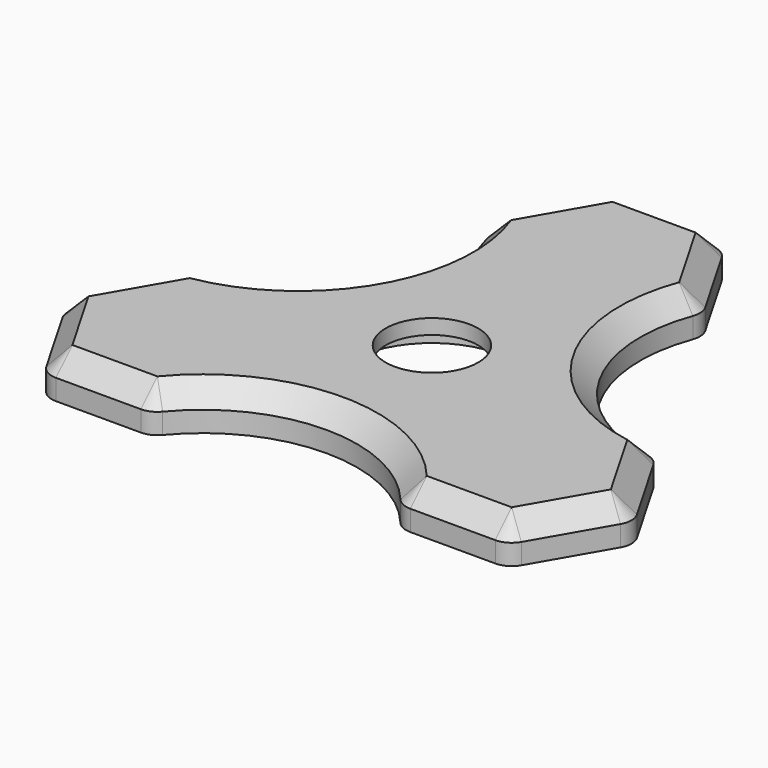
from build123d import *

# Parameters (mm, degrees)
F1_DEPTH = 4
F2_R     = 8.075
F3_DEPTH = 2.55
F5_DEPTH = 3.2
F6_SIZE  = 1.99999
F7_R     = 4.5
F8_DEPTH = 25


# Not quite as in the source:
# - a fillet or chamfer is up to 0.001 mm smaller than in the source, because OpenCascade refuses the exact size


with BuildPart() as f1:
    # F0 (on Top) → F1 (new body)
    with BuildSketch(Plane.XY):
        with BuildLine():
            Line((-5.7735026919, 28), (-9.9042445516, 20.8453452261))
            ThreePointArc((-9.9042445516, 20.8453452261), (-10.1650850266, 20.0138217399), (-10.0475406836, 19.1503100787))
            ThreePointArc((-10.0475406836, 19.1503100787), (-11.1235598668, 6.4221902835), (-21.6084253603, -0.8737295618))
            ThreePointArc((-21.6084253603, -0.8737295618), (-22.4150205669, -1.2036890053), (-23.0047207922, -1.8453452261))
            Line((-23.0047207922, -1.8453452261), (-27.1354626519, -9))
            ThreePointArc((-27.1354626519, -9), (-27.4034118443, -10), (-27.1354626519, -11))
            Line((-27.1354626519, -11), (-23.0940107676, -18))
            ThreePointArc((-23.0940107676, -18), (-22.36195996, -18.7320508076), (-21.36195996, -19))
            Line((-21.36195996, -19), (-13.1004762407, -19))
            ThreePointArc((-13.1004762407, -19), (-12.2499355402, -18.8101327346), (-11.5608846767, -18.2765805169))
            ThreePointArc((-11.5608846767, -18.2765805169), (0, -12.8443805669), (11.5608846767, -18.2765805169))
            ThreePointArc((11.5608846767, -18.2765805169), (12.2499355402, -18.8101327346), (13.1004762407, -19))
            Line((13.1004762407, -19), (21.36195996, -19))
            ThreePointArc((21.36195996, -19), (22.36195996, -18.7320508076), (23.0940107676, -18))
            Line((23.0940107676, -18), (27.1354626519, -11))
            ThreePointArc((27.1354626519, -11), (27.4034118443, -10), (27.1354626519, -9))
            Line((27.1354626519, -9), (23.0047207922, -1.8453452261))
            ThreePointArc((23.0047207922, -1.8453452261), (22.4150205669, -1.2036890053), (21.6084253603, -0.8737295618))
            ThreePointArc((21.6084253603, -0.8737295618), (11.1235598668, 6.4221902835), (10.0475406836, 19.1503100787))
            ThreePointArc((10.0475406836, 19.1503100787), (10.1650850266, 20.0138217399), (9.9042445516, 20.8453452261))
            Line((9.9042445516, 20.8453452261), (5.7735026919, 28))
            ThreePointArc((5.7735026919, 28), (5.0414518843, 28.7320508076), (4.0414518843, 29))
            Line((4.0414518843, 29), (-4.0414518843, 29))
            ThreePointArc((-4.0414518843, 29), (-5.0414518843, 28.7320508076), (-5.7735026919, 28))
        make_face()
    extrude(amount=F1_DEPTH)

    # F2 (on face) → F3 (cut)
    with BuildSketch(Plane.XY):
        Circle(F2_R)
    extrude(amount=F3_DEPTH, mode=Mode.SUBTRACT)

    # F4 (on face) → F5 (cut)
    with BuildSketch(Plane.XY):
        Polygon((6.9282032303, 20), (3.4641016151, 26), (-3.4641016151, 26), (-6.9282032303, 20), (-3.4641016151, 14), (3.4641016151, 14), align=None)
        Polygon((-13.8564064606, -16), (-10.3923048454, -10), (-13.8564064606, -4), (-20.7846096908, -4), (-24.248711306, -10), (-20.7846096908, -16), align=None)
        Polygon((20.7846096908, -4), (13.8564064606, -4), (10.3923048454, -10), (13.8564064606, -16), (20.7846096908, -16), (24.248711306, -10), align=None)
    extrude(amount=F5_DEPTH, mode=Mode.SUBTRACT)

    # F6 (size 2 in the source; OpenCascade refuses exactly that, so slightly less here)
    f6_edges = [f1.edges().sort_by_distance(p)[0] for p in [
        (10.165085, 20.013822, 4),
        (7.838874, 24.422673, 4),
        (5.041452, 28.732051, 4),
        (0, 29, 4),
        (-5.041452, 28.732051, 4),
        (-7.838874, 24.422673, 4),
        (-10.165085, 20.013822, 4),
        (-11.12356, 6.42219, 4),
        (-22.415021, -1.203689, 4),
        (-25.070092, -5.422673, 4),
        (-27.403412, -10, 4),
        (-25.114737, -14.5, 4),
        (-22.36196, -18.732051, 4),
        (-17.231218, -19, 4),
        (-12.249936, -18.810133, 4),
        (0, -12.844381, 4),
        (12.249936, -18.810133, 4),
        (17.231218, -19, 4),
        (22.36196, -18.732051, 4),
        (25.114737, -14.5, 4),
        (27.403412, -10, 4),
        (25.070092, -5.422673, 4),
        (22.415021, -1.203689, 4),
        (11.12356, 6.42219, 4),
    ]]
    chamfer(f6_edges, length=F6_SIZE)

    # F7 (on face) → F8 (cut)
    with BuildSketch(Plane.XY.offset(4)):
        Circle(F7_R)
    extrude(amount=-F8_DEPTH, mode=Mode.SUBTRACT)


solid = f1.part
